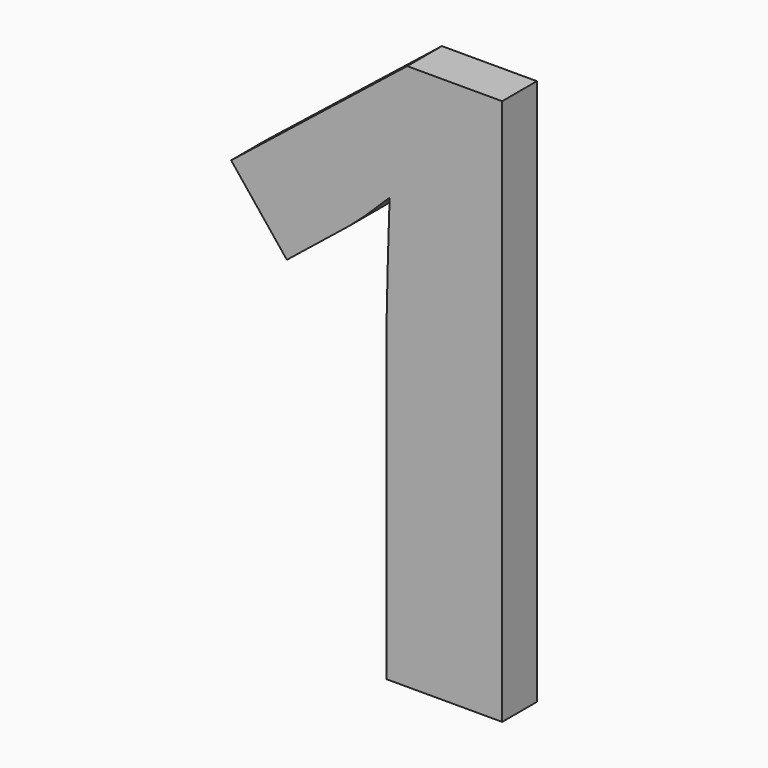
from build123d import *

# Parameters (mm, degrees)
F0_TEXT_SIZE = 70.5555555556
F1_DEPTH     = 4


# Not quite as in the source:
# - Text() gives the source's letters only with a copy of the font that has no kerning and outlines rounded to 1/6400 em; it was checked with that copy


with BuildPart() as f1:
    # F0 (on Front) → F1 (new body)
    with BuildSketch(Plane.XZ):
        with Locations((0, 0)):
            Text('1', F0_TEXT_SIZE, font='Open Sans', font_style=FontStyle.BOLD, text_align=(TextAlign.LEFT, TextAlign.BOTTOM))
    extrude(amount=F1_DEPTH)


solid = f1.part
